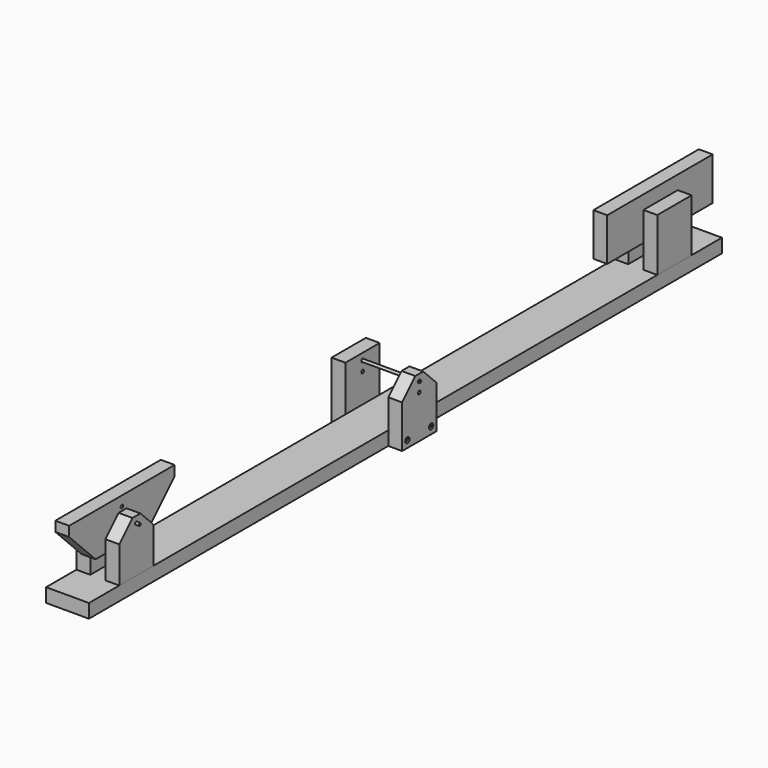
from build123d import *

# Parameters (mm, degrees)
F0_W              = 65
F0_H              = 1200
F1_DEPTH          = 21
F2_W              = 21
F2_H              = 65
F3_DEPTH          = 80
F4_W              = 200
F4_H              = 65
F5_DEPTH          = 10.5
F7_D              = 5
F8_D              = 5
F9_W              = 21
F9_H              = 65
F10_DEPTH         = 90
F12_D             = 5
F12_2_D           = 5
F13_SIZE          = 25
F13_2_SIZE        = 25
F15_D             = 5
F15_DEPTH         = 25
F15_CSINK_D       = 8.3
F15_CSINK_ANGLE   = 90
F15_TIP           = 1.5021515476
F15_2_D           = 5
F15_2_DEPTH       = 25
F15_2_CSINK_D     = 8.3
F15_2_CSINK_ANGLE = 90
F15_2_TIP         = 1.5021515476
F15_3_D           = 5
F15_3_DEPTH       = 25
F15_3_CSINK_D     = 8.3
F15_3_CSINK_ANGLE = 90
F15_3_TIP         = 1.5021515476
F15_4_D           = 5
F15_4_DEPTH       = 25
F15_4_CSINK_D     = 8.3
F15_4_CSINK_ANGLE = 90
F15_4_TIP         = 1.5021515476
F15_5_D           = 5
F15_5_DEPTH       = 25
F15_5_CSINK_D     = 8.3
F15_5_CSINK_ANGLE = 90
F15_5_TIP         = 1.5021515476
F17_D             = 5
F17_DEPTH         = 25
F17_CSINK_D       = 8.3
F17_CSINK_ANGLE   = 90
F17_TIP           = 1.5021515476
F17_2_D           = 5
F17_2_DEPTH       = 25
F17_2_CSINK_D     = 8.3
F17_2_CSINK_ANGLE = 90
F17_2_TIP         = 1.5021515476
F18_R             = 2
F19_DEPTH         = 55
F20_R             = 2
F21_DEPTH         = 37.5
F22_SIZE          = 50


# Not quite as in the source:
# - a feature names something its author has since deleted; it is built from what else it names


with BuildPart() as f1:
    # F0 (on Top) → F1 (new body)
    with BuildSketch(Plane.XY):
        Rectangle(F0_W, F0_H)
    extrude(amount=F1_DEPTH)

    # F15
    with Locations(Plane(origin=(0, 0, 0), x_dir=(1, 0, 0), z_dir=(0, 0, -1))):
        with Locations((22, -487.5), (22, -532.5), (-22, -487.5), (-22, -532.5), (22, 532.5), (22, 487.5), (-22, 532.5), (-22, 487.5)):
            CounterSinkHole(F15_D / 2, F15_CSINK_D / 2, depth=F15_DEPTH, counter_sink_angle=F15_CSINK_ANGLE)
            with Locations((0, 0, -(F15_DEPTH + F15_TIP / 2))):  # 118° drill point
                Cone(0, F15_D / 2, F15_TIP, mode=Mode.SUBTRACT)

    # F17
    with Locations(Plane.YZ.offset(53.5)):
        with Locations((-22.5, 10.5), (22.5, 10.5)):
            CounterSinkHole(F17_D / 2, F17_CSINK_D / 2, depth=F17_DEPTH, counter_sink_angle=F17_CSINK_ANGLE)
            with Locations((0, 0, -(F17_DEPTH + F17_TIP / 2))):  # 118° drill point
                Cone(0, F17_D / 2, F17_TIP, mode=Mode.SUBTRACT)


with BuildPart() as f3:
    # F2 (on face) → F3 (new body)
    with BuildSketch(Plane.XY.offset(21)):
        with Locations((-22, 510)):
            Rectangle(F2_W, F2_H)
    extrude(amount=F3_DEPTH)

    # F15#2
    with Locations(Plane(origin=(0, 0, 0), x_dir=(1, 0, 0), z_dir=(0, 0, -1))):
        with Locations((22, -487.5), (22, -532.5), (-22, -487.5), (-22, -532.5), (22, 532.5), (22, 487.5), (-22, 532.5), (-22, 487.5)):
            CounterSinkHole(F15_2_D / 2, F15_2_CSINK_D / 2, depth=F15_2_DEPTH, counter_sink_angle=F15_2_CSINK_ANGLE)
            with Locations((0, 0, -(F15_2_DEPTH + F15_2_TIP / 2))):  # 118° drill point
                Cone(0, F15_2_D / 2, F15_2_TIP, mode=Mode.SUBTRACT)


with BuildPart() as f3b:
    # F2 (on face) → F3, piece 2 (new body)
    with BuildSketch(Plane.XY.offset(21)):
        with Locations((-22, -510)):
            Rectangle(F2_W, F2_H)
    extrude(amount=F3_DEPTH)

    # F15#3
    with Locations(Plane(origin=(0, 0, 0), x_dir=(1, 0, 0), z_dir=(0, 0, -1))):
        with Locations((22, -487.5), (22, -532.5), (-22, -487.5), (-22, -532.5), (22, 532.5), (22, 487.5), (-22, 532.5), (-22, 487.5)):
            CounterSinkHole(F15_3_D / 2, F15_3_CSINK_D / 2, depth=F15_3_DEPTH, counter_sink_angle=F15_3_CSINK_ANGLE)
            with Locations((0, 0, -(F15_3_DEPTH + F15_3_TIP / 2))):  # 118° drill point
                Cone(0, F15_3_D / 2, F15_3_TIP, mode=Mode.SUBTRACT)


with BuildPart() as f3c:
    # F2 (on face) → F3, piece 3 (new body)
    with BuildSketch(Plane.XY.offset(21)):
        with Locations((22, 510)):
            Rectangle(F2_W, F2_H)
    extrude(amount=F3_DEPTH)

    # F15#4
    with Locations(Plane(origin=(0, 0, 0), x_dir=(1, 0, 0), z_dir=(0, 0, -1))):
        with Locations((22, -487.5), (22, -532.5), (-22, -487.5), (-22, -532.5), (22, 532.5), (22, 487.5), (-22, 532.5), (-22, 487.5)):
            CounterSinkHole(F15_4_D / 2, F15_4_CSINK_D / 2, depth=F15_4_DEPTH, counter_sink_angle=F15_4_CSINK_ANGLE)
            with Locations((0, 0, -(F15_4_DEPTH + F15_4_TIP / 2))):  # 118° drill point
                Cone(0, F15_4_D / 2, F15_4_TIP, mode=Mode.SUBTRACT)


with BuildPart() as f3d:
    # F2 (on face) → F3, piece 4 (new body)
    with BuildSketch(Plane.XY.offset(21)):
        with Locations((22, -510)):
            Rectangle(F2_W, F2_H)
    extrude(amount=F3_DEPTH)

    # F7 (through all)
    with Locations(Plane.YZ.offset(32.5)):
        with Locations((-510, 91)):
            Hole(F7_D / 2)

    # F13
    f13_edges = [f3d.edges().sort_by_distance(p)[0] for p in [
        (22, -542.5, 101),
        (22, -477.5, 101),
    ]]
    chamfer(f13_edges, length=F13_SIZE)

    # F15#5
    with Locations(Plane(origin=(0, 0, 0), x_dir=(1, 0, 0), z_dir=(0, 0, -1))):
        with Locations((22, -487.5), (22, -532.5), (-22, -487.5), (-22, -532.5), (22, 532.5), (22, 487.5), (-22, 532.5), (-22, 487.5)):
            CounterSinkHole(F15_5_D / 2, F15_5_CSINK_D / 2, depth=F15_5_DEPTH, counter_sink_angle=F15_5_CSINK_ANGLE)
            with Locations((0, 0, -(F15_5_DEPTH + F15_5_TIP / 2))):  # 118° drill point
                Cone(0, F15_5_D / 2, F15_5_TIP, mode=Mode.SUBTRACT)


with BuildPart() as f5:
    # F4 (on Right) → F5 (new body, symmetric)
    with BuildSketch(Plane.YZ):
        with Locations((-510, 88.5)):
            Rectangle(F4_W, F4_H)
    extrude(amount=F5_DEPTH, both=True)

    # F8 (through all)
    with Locations(Plane.YZ.offset(32.5)):
        with Locations((-510, 76), (-510, 91), (-510, 106)):
            Hole(F8_D / 2)

    # F22
    f22_edges = [f5.edges().sort_by_distance(p)[0] for p in [
        (0, -610, 56),
        (0, -410, 56),
    ]]
    chamfer(f22_edges, length=F22_SIZE)


with BuildPart() as f5b:
    # F4 (on Right) → F5, piece 2 (new body, symmetric)
    with BuildSketch(Plane.YZ):
        with Locations((510, 88.5)):
            Rectangle(F4_W, F4_H)
    extrude(amount=F5_DEPTH, both=True)


with BuildPart() as f10:
    # F9 (on Top) → F10 (new body)
    with BuildSketch(Plane.XY):
        with Locations((-43, 0)):
            Rectangle(F9_W, F9_H)
    extrude(amount=F10_DEPTH)

    # F12 (through all)
    with Locations(Plane.YZ.offset(53.5)):
        with Locations((0, 80), (0, 65)):
            Hole(F12_D / 2)


with BuildPart() as f10b:
    # F9 (on Top) → F10, piece 2 (new body)
    with BuildSketch(Plane.XY):
        with Locations((43, 0)):
            Rectangle(F9_W, F9_H)
    extrude(amount=F10_DEPTH)

    # F12#2 (through all)
    with Locations(Plane.YZ.offset(53.5)):
        with Locations((0, 80), (0, 65)):
            Hole(F12_2_D / 2)

    # F13#2
    f13_2_edges = [f10b.edges().sort_by_distance(p)[0] for p in [
        (43, -32.5, 90),
        (43, 32.5, 90),
    ]]
    chamfer(f13_2_edges, length=F13_2_SIZE)

    # F17#2
    with Locations(Plane.YZ.offset(53.5)):
        with Locations((-22.5, 10.5), (22.5, 10.5)):
            CounterSinkHole(F17_2_D / 2, F17_2_CSINK_D / 2, depth=F17_2_DEPTH, counter_sink_angle=F17_2_CSINK_ANGLE)
            with Locations((0, 0, -(F17_2_DEPTH + F17_2_TIP / 2))):  # 118° drill point
                Cone(0, F17_2_D / 2, F17_2_TIP, mode=Mode.SUBTRACT)


with BuildPart() as f19:
    # F18 (on Right) → F19 (new body, symmetric)
    with BuildSketch(Plane.YZ):
        with Locations((0, 80)):
            Circle(F18_R)
    extrude(amount=F19_DEPTH, both=True)


with BuildPart() as f21:
    # F20 (on Right) → F21 (new body, symmetric)
    with BuildSketch(Plane.YZ):
        with Locations((-510, 91)):
            Circle(F20_R)
    extrude(amount=F21_DEPTH, both=True)


solid = Compound([f1.part, f3.part, f3b.part, f3c.part, f3d.part, f5.part, f5b.part, f10.part, f10b.part, f19.part, f21.part])
